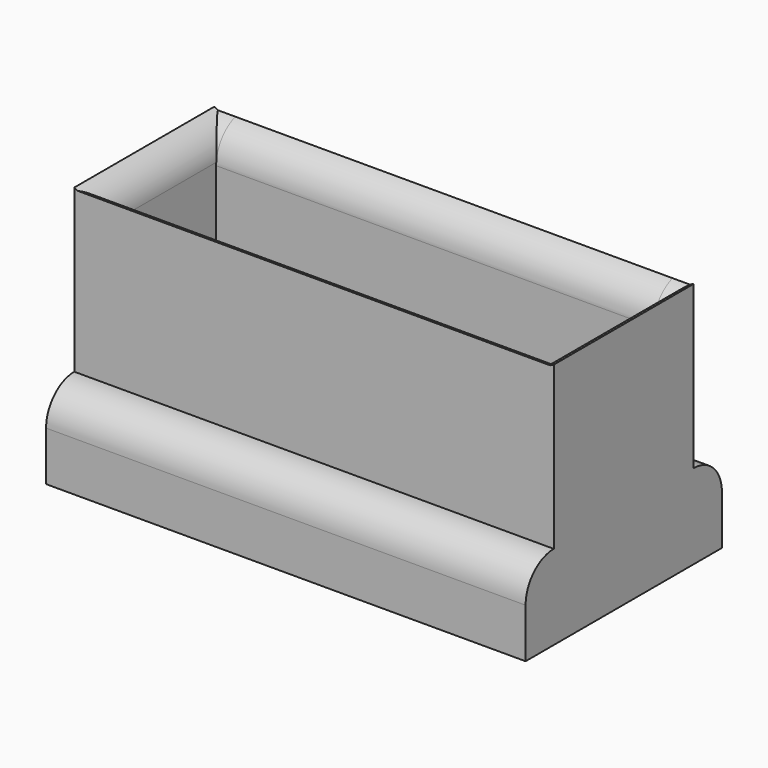
from build123d import *

# Parameters (mm, degrees)
F0_W         = 68
F0_H         = 24.8
F0_W_2       = 62
F0_H_2       = 18
F1_DEPTH     = 35
F0_H_3       = 5
F2_DEPTH     = 12
F3_R         = 6.7597979746
F4_R         = 6.7597979746
F5_R         = 4.99999
F6_R         = 4.99999
F7_T1_DEPTH  = 62
F8_T1_DEPTH  = 62
F9_T4_DEPTH  = 47.7128784748
F9_S5_R      = 5.0000000001
F9_T6_DEPTH  = 26
F9_S7_R      = 5.0000000001
F9_T8_DEPTH  = 26
F10_T4_DEPTH = 47.7128784748
F10_S5_R     = 5.0000000001
F10_T6_DEPTH = 26
F10_S7_R     = 5.0000000001
F10_T8_DEPTH = 26


# Not quite as in the source:
# - a fillet or chamfer that OpenCascade refuses, or shapes differently, is made with other operations: its cross-section is extruded or revolved along the edge and cut away or added
# - a fillet or chamfer is up to 0.001 mm smaller than in the source, because OpenCascade refuses the exact size


with BuildPart() as f1:
    # F0 (on Top) → F1 (new body)
    with BuildSketch(Plane.XY):
        Rectangle(F0_W, F0_H)
        Rectangle(F0_W_2, F0_H_2, mode=Mode.SUBTRACT)
    extrude(amount=F1_DEPTH)

    # F0 (on Top) → F2 (join)
    with BuildSketch(Plane.XY):
        with Locations((0, 14.9)):
            Rectangle(F0_W, F0_H_3)
        with Locations((0, -14.9)):
            Rectangle(F0_W, F0_H_3)
    extrude(amount=F2_DEPTH)

    # F3
    f3_edges = [f1.edges().sort_by_distance(p)[0] for p in [
        (0, 9, 0),
    ]]
    fillet(f3_edges, radius=F3_R)

    # F4
    f4_edges = [f1.edges().sort_by_distance(p)[0] for p in [
        (0, -9, 0),
    ]]
    fillet(f4_edges, radius=F4_R)

    # F5 (radius 5 in the source; OpenCascade refuses exactly that, so slightly less here)
    f5_edges = [f1.edges().sort_by_distance(p)[0] for p in [
        (0, 17.4, 12),
    ]]
    fillet(f5_edges, radius=F5_R)

    # F6 (radius 5 in the source; OpenCascade refuses exactly that, so slightly less here)
    f6_edges = [f1.edges().sort_by_distance(p)[0] for p in [
        (0, -17.4, 12),
    ]]
    fillet(f6_edges, radius=F6_R)

    # F7: fillet of radius 5 on 1 edges, made by hand

    # F7_s2 → F7_t1 (cut)
    with BuildSketch(Plane.YZ.offset(-31)):
        with BuildLine():
            ThreePointArc((14, 35), (10.4644660941, 33.5355339059), (9, 30))
            Line((9, 30), (9, 35))
            Line((9, 35), (14, 35))
        make_face()
    extrude(amount=F7_T1_DEPTH, mode=Mode.SUBTRACT)

    # F8: fillet of radius 5 on 1 edges, made by hand

    # F8_s2 → F8_t1 (cut)
    with BuildSketch(Plane.YZ.offset(-31)):
        with BuildLine():
            ThreePointArc((-9, 30), (-10.4644660941, 33.5355339059), (-14, 35))
            Line((-14, 35), (-9, 35))
            Line((-9, 35), (-9, 30))
        make_face()
    extrude(amount=F8_T1_DEPTH, mode=Mode.SUBTRACT)

    # F9: fillet of radius 5 on 1 edges, made by hand


with BuildPart() as f9_tool2:
    # F9_s3 → F9_t4 (new body)
    with BuildSketch(Plane.XZ.offset(-23.8564392374)):
        with BuildLine():
            ThreePointArc((-31, 30.417424305), (-31.8166998673, 33.1560370926), (-34, 35))
            Line((-34, 35), (-31, 35))
            Line((-31, 35), (-31, 30.417424305))
        make_face()
    extrude(amount=F9_T4_DEPTH)

    # F9_s5 → F9_t6 (cut, symmetric)
    with BuildSketch(Plane.YZ.offset(-32.5)):
        with Locations((-14.0000000001, 29.9999999999)):
            Circle(F9_S5_R)
    extrude(amount=F9_T6_DEPTH, both=True, mode=Mode.SUBTRACT)

    # F9_s7 → F9_t8 (cut, symmetric)
    with BuildSketch(Plane.YZ.offset(-32.5)):
        with Locations((14.0000000001, 29.9999999999)):
            Circle(F9_S7_R)
    extrude(amount=F9_T8_DEPTH, both=True, mode=Mode.SUBTRACT)


with BuildPart() as f1_1:
    add(f1.part)

    # F9_t1: cut F9_tool2
    add(f9_tool2.part, mode=Mode.SUBTRACT)

    # F10: fillet of radius 5 on 1 edges, made by hand


with BuildPart() as f10_tool2:
    # F10_s3 → F10_t4 (new body)
    with BuildSketch(Plane.XZ.offset(-23.8564392374)):
        with BuildLine():
            ThreePointArc((31, 30.417424305), (31.8166998673, 33.1560370926), (34, 35))
            Line((34, 35), (31, 35))
            Line((31, 35), (31, 30.417424305))
        make_face()
    extrude(amount=F10_T4_DEPTH)

    # F10_s5 → F10_t6 (cut, symmetric)
    with BuildSketch(Plane.YZ.offset(32.5)):
        with Locations((-14.0000000001, 29.9999999999)):
            Circle(F10_S5_R)
    extrude(amount=F10_T6_DEPTH, both=True, mode=Mode.SUBTRACT)

    # F10_s7 → F10_t8 (cut, symmetric)
    with BuildSketch(Plane.YZ.offset(32.5)):
        with Locations((14.0000000001, 29.9999999999)):
            Circle(F10_S7_R)
    extrude(amount=F10_T8_DEPTH, both=True, mode=Mode.SUBTRACT)


with BuildPart() as f1_2:
    add(f1_1.part)

    # F10_t1: cut F10_tool2
    add(f10_tool2.part, mode=Mode.SUBTRACT)


solid = f1_2.part
